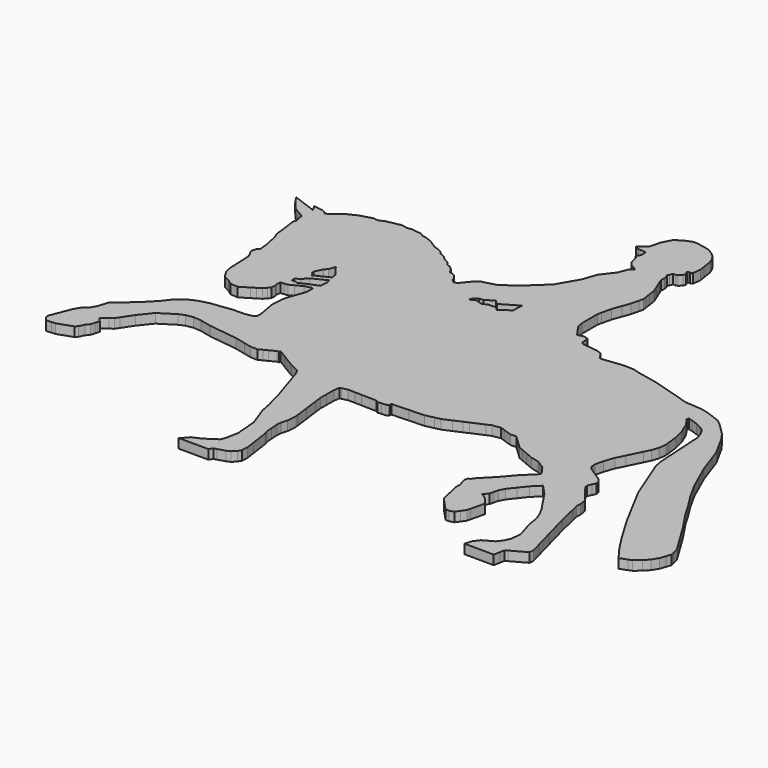
from build123d import *

# Parameters (mm, degrees)
F1_DEPTH = 6.35
F2_SCALE = 0.85


# Not quite as in the source:
# - ends of sketch curves that miss each other by under 0.0002 mm in the source are joined


with BuildPart() as f1:
    # F0 (on Top) → F1 (new body)
    with BuildSketch(Plane.XY):
        Polygon((-13.5594852, 161.1981282), (-15.3749502, 153.9993872), (-17.5161448, 152.6285238), (-20.7511396, 149.630257), (-18.0455062, 148.39569), (-12.6456948, 147.858353), (-12.6219966, 147.147788), (-12.5753876, 145.7501784), (-12.5165612, 143.986504), (-13.7517632, 142.1640286), (-14.1046708, 140.9294616), (-12.911709, 140.0959606), (-12.697206, 139.238355), (-12.2184922, 137.3244142), (-11.4538506, 134.2673718), (-9.3327474, 131.4925488), (-6.5719198, 130.034538), (-4.747133, 129.070862), (-5.6896508, 128.3296646), (-7.3535286, 127.0211836), (-8.5178646, 124.0731326), (-10.0039678, 120.3103004), (-12.3753626, 117.2887926), (-14.3408654, 114.7844288), (-16.4336984, 112.1178606), (-18.105247, 107.3182004), (-19.8354696, 102.3500366), (-23.1120442, 96.7057756), (-27.8045418, 88.6224542), (-31.3029346, 85.3369896), (-40.0668744, 77.1065006), (-50.4377452, 69.6153294), (-54.205886, 68.6302666), (-59.3993478, 67.2725604), (-62.914403, 64.9672056), (-65.692909, 61.5112308), (-68.3397414, 58.2190352), (-70.5160134, 57.337198), (-72.8844364, 59.4073234), (-73.4137978, 61.2885744), (-75.1195348, 63.6401318), (-77.8251682, 65.0510764), (-79.5897316, 65.4038316), (-81.0095662, 68.1746414), (-83.2446646, 70.173469), (-85.5973904, 71.1141072), (-87.1855, 73.1717358), (-90.617294, 74.9848132), (-91.067509, 75.4057166), (-92.902786, 77.1215374), (-96.8436214, 79.0027884), (-97.667064, 80.2373808), (-101.2549918, 82.1186318), (-103.7253704, 82.8240914), (-109.976412, 86.8835956), (-114.0937012, 88.3533158), (-116.6228808, 88.7648466), (-118.9168056, 90.2933678), (-126.0926358, 91.175205), (-128.5630144, 90.7048986), (-132.8142886, 91.5578306), (-136.8693732, 90.7192496), (-139.5204474, 90.171016), (-142.9319214, 89.4655564), (-146.033617, 87.949405), (-147.2354434, 88.046814), (-149.7287074, 88.2489472), (-153.4701782, 87.1649768), (-157.528641, 85.9892108), (-164.1585236, 82.827876), (-166.1786618, 81.272888), (-171.2958728, 77.3340084), (-173.1780636, 76.3345946), (-174.4132402, 77.7455392), (-176.8247924, 78.6861774), (-182.8242724, 79.6855912), (-180.4715212, 75.629135), (-196.5877704, 81.5668422), (-192.9998426, 76.3345946), (-188.2943656, 70.9259948), (-180.8160976, 66.625216), (-180.52161, 63.493523), (-179.698142, 61.6710476), (-180.3883108, 58.723657), (-179.9922486, 55.6745394), (-178.6976106, 45.707681), (-178.5211314, 43.0033684), (-176.7565934, 38.1826516), (-174.9891598, 29.5782492), (-174.3421456, 23.4641644), (-175.8714288, 21.759291), (-176.8125242, 18.7022486), (-173.9942164, 13.167614), (-173.8757254, 10.4908858), (-173.572043, 3.6312094), (-173.2779364, -3.0119828), (-172.4848468, -7.733919), (-170.7487568, -10.5370122), (-169.2194736, -13.0061462), (-165.3238502, -14.8990304), (-161.9123762, -17.485741), (-156.7532552, -17.8927506), (-150.9220502, -14.3583914), (-148.0312508, -12.6062486), (-145.3319928, -10.9701838), (-143.6198804, -8.9613232), (-142.267051, -7.374001), (-141.9729444, -4.5521118), (-142.5023312, -2.7296618), (-142.1407114, 0.0580898), (-139.7966724, 0.3273806), (-137.3711756, 0.606044), (-134.2089264, 2.2674326), (-129.6211022, 4.677791), (-125.033278, 5.7947814), (-124.20981, 5.4420516), (-124.5156006, 0.0899668), (-126.978664, -6.9225922), (-128.9196812, -12.4487686), (-129.8023058, -21.8769184), (-127.5066538, -35.0687894), (-127.6831076, -37.6555254), (-129.3300182, -39.007669), (-134.682484, -39.8895062), (-142.5683712, -40.0267678), (-148.3478364, -40.7748232), (-156.5235884, -41.833038), (-162.2289618, -43.3027582), (-166.6403322, -45.0664326), (-170.22826, -47.2416378), (-174.2867228, -50.710211), (-178.2987036, -55.8449226), (-184.8863714, -62.723268), (-193.3650692, -70.3360544), (-198.4905098, -74.3402374), (-199.3057228, -76.9204456), (-200.7173532, -81.3884326), (-203.0789944, -85.5258894), (-206.431642, -88.4065542), (-208.798033, -92.3547302), (-211.19592, -98.4595186), (-214.3132874, -106.3960788), (-214.19566, -108.2185288), (-211.7847682, -111.206915), (-208.3726592, -110.9816424), (-205.5935944, -110.7981528), (-195.653279, -107.2707786), (-194.2326316, -105.7961054), (-192.585721, -102.3275322), (-190.6311402, -99.917504), (-189.8298972, -97.3421726), (-189.3507008, -95.801942), (-188.9049054, -94.369001), (-189.7036084, -93.4503592), (-191.4109202, -91.4866852), (-187.4030796, -88.4413776), (-185.1084436, -86.69782), (-183.3985664, -84.1324962), (-178.5717028, -76.8906514), (-171.9197984, -68.5932842), (-161.61512, -62.0641126), (-158.0271922, -60.4768158), (-153.2629142, -59.6537542), (-147.7927956, -60.065285), (-140.1283456, -61.8401354), (-120.6822326, -64.2982966), (-113.6962166, -65.9645874), (-108.5202046, -67.1991544), (-103.819579, -67.2790628), (-101.1929904, -65.9473916), (-98.4452946, -64.5543286), (-94.3868318, -62.4967), (-93.0928288, -62.4379244), (-92.7708584, -61.3130092), (-86.8513122, -64.9144244), (-78.7343866, -69.8527178), (-72.2020146, -73.1011238), (-70.6466202, -75.7986546), (-67.0811206, -86.8151426), (-62.3731036, -101.3617734), (-59.1379818, -113.8447812), (-57.9923148, -120.0834022), (-54.3089592, -130.1536386), (-52.9630132, -133.8334382), (-52.5443958, -138.8544594), (-51.7358122, -148.5531446), (-52.5432782, -152.6360168), (-53.5432, -157.6918868), (-54.6103302, -160.1483462), (-57.2334136, -161.8852236), (-59.601481, -163.4532418), (-62.5777768, -165.4240024), (-65.4833336, -166.6866618), (-68.188967, -167.8624278), (-70.0711578, -169.8024798), (-70.8357994, -171.2134244), (-72.1886288, -171.918884), (-72.8356176, -172.7419456), (-52.5753838, -172.7960222), (-51.0100834, -170.5091332), (-49.0462824, -169.9153574), (-44.1587636, -168.43756), (-41.5707576, -167.2617686), (-39.2153648, -164.8360432), (-37.9213618, -162.660838), (-37.6275346, -158.512129), (-38.5710176, -151.8843292), (-40.2222716, -140.2848858), (-41.1129734, -137.546715), (-41.3986472, -133.4065404), (-41.7515548, -128.2918694), (-41.5762948, -125.0391962), (-40.2822918, -120.923939), (-39.8046194, -114.6921252), (-40.0651218, -112.6588552), (-41.2047436, -103.764334), (-42.3415968, -94.8914536), (-42.9747934, -89.9495534), (-42.9297846, -84.9560658), (-42.8709582, -78.4304502), (-42.2566338, -74.5899702), (-41.1064202, -74.3152184), (-37.3378984, -73.4149916), (-32.6724518, -73.5141786), (-28.145486, -73.6104192), (-17.7279554, -73.8318818), (-17.4853346, -74.0242614), (-16.45666, -74.8400332), (-13.720953, -74.6121698), (-10.8976922, -74.3769912), (-9.368409, -73.495154), (-9.0692986, -71.9237068), (2.2961092, -71.495539), (12.4181616, -71.1142088), (18.1943756, -69.8443866), (22.0813122, -68.9899052), (27.76601, -66.4898848), (32.939482, -64.2146798), (36.3673136, -62.7071898), (44.6301114, -59.0733642), (47.571025, -57.7799962), (53.1573486, -56.9123068), (55.8745644, -57.8450202), (61.6975906, -59.8438478), (65.569719, -59.6190578), (66.2569414, -60.2732856), (68.4092358, -62.322202), (74.9568986, -68.5553874), (77.6381734, -69.674486), (81.88833, -71.4483966), (87.2407958, -73.6823774), (92.647262, -74.9761264), (95.4165478, -76.6806442), (98.2669612, -78.4350984), (99.777804, -80.516603), (101.9541014, -83.5148444), (102.6673334, -85.4077032), (101.7776476, -86.2779326), (94.2413152, -93.6494952), (86.9478322, -102.1151374), (78.9430222, -110.3117428), (76.8255512, -113.133632), (75.9811282, -113.0547396), (75.649201, -114.1330458), (75.1786406, -115.661567), (77.1196578, -122.2459582), (76.6021328, -123.4571572), (78.8841958, -134.062597), (79.9635942, -139.078843), (80.8085506, -139.9872486), (81.2150776, -140.4243318), (83.2315328, -142.5922218), (86.1869752, -145.7696348), (88.5441968, -148.3038944), (91.0734018, -148.36267), (93.9496216, -147.4582268), (95.8965062, -144.7177446), (97.9189812, -141.8708364), (98.4967042, -139.4701046), (100.7802658, -129.9807662), (99.6133898, -128.5154148), (97.3194904, -125.63475), (93.6708058, -123.0925656), (92.7147752, -122.6612736), (93.3767246, -121.9167742), (95.3337438, -119.715661), (95.9059042, -117.3900116), (96.7881732, -113.8038618), (98.6735898, -110.2226396), (102.493572, -105.3969952), (106.7284886, -100.047171), (111.9280718, -94.9476638), (114.0244608, -97.1812636), (118.142512, -101.568885), (123.7943168, -110.0118958), (128.3279374, -116.7845264), (130.798316, -121.4288656), (132.7393332, -126.6023122), (133.9188584, -134.093458), (137.4859074, -145.926429), (137.0386134, -149.6946206), (136.6268794, -153.1631938), (134.803515, -157.0432724), (132.278501, -160.282636), (128.804035, -162.27552), (125.0928918, -164.404167), (124.039757, -165.8616698), (122.3109822, -168.2542482), (121.451751, -171.152693), (120.9811906, -172.7400152), (140.876909, -172.893482), (141.647291, -168.6630358), (142.2295606, -165.4655822), (143.8823894, -164.547804), (153.9403322, -158.9628266), (154.2497296, -155.9990022), (152.3248414, -148.8355672), (148.6990422, -135.3422236), (144.2629576, -118.8333666), (141.4003014, -106.378502), (140.4003796, -102.0280916), (140.5951468, -99.0048312), (140.1629404, -96.4833986), (139.7758698, -94.2253132), (136.338564, -89.83726), (130.3979104, -82.253455), (130.0159706, -80.260952), (131.2779188, -77.5280898), (132.3366416, -75.235308), (132.0425604, -72.9425262), (129.9662374, -70.5225666), (125.6313464, -67.710304), (120.1579512, -64.1594094), (118.3345868, -61.749051), (118.0993066, -58.574432), (119.3933096, -52.9894546), (121.7419968, -46.347126), (124.580523, -40.5940514), (129.105533, -31.4229242), (131.2229786, -27.1313148), (132.7522618, -22.6045268), (133.3612522, -17.6188624), (133.0468256, -14.9502114), (132.2212748, -7.9437738), (130.5054794, -0.8137906), (128.9862546, 2.8734258), (127.4524756, 6.5959736), (125.0454192, 10.104501), (123.6337888, 12.1621296), (124.0930716, 13.4510018), (126.6923298, 12.632436), (130.9860728, 11.2802924), (135.5739224, 8.9875106), (137.8166916, 7.0895972), (140.110591, 3.2683196), (141.3658844, -0.9285478), (141.5890488, -4.75742), (142.0390098, -12.4779532), (142.9332168, -27.821001), (143.2861498, -33.8762848), (144.3800516, -39.845361), (148.819743, -51.0711958), (156.1292026, -69.5532772), (164.4222518, -85.1556336), (171.3700916, -98.2271086), (181.7329106, -115.592987), (187.9088444, -125.2344206), (194.9733464, -134.810119), (199.848978, -132.9358022), (202.1429028, -132.053965), (206.3217616, -128.573784), (209.439129, -125.2815884), (211.967191, -121.1609972), (213.2169472, -117.4032704), (214.3132874, -114.1068076), (213.7388664, -111.5767898), (212.8828102, -107.806236), (208.6443884, -100.8661178), (199.5825066, -86.027895), (197.2842384, -82.5810134), (191.0201666, -73.1863408), (187.0080842, -66.2111452), (180.745638, -56.319039), (174.3556838, -44.7984626), (170.5052216, -36.1900724), (166.169975, -26.497915), (162.0055942, -14.6172428), (159.5699374, -7.6684886), (158.4496196, -5.6369458), (156.0258754, -1.2418568), (154.554555, 1.4261846), (151.9164602, 6.2099444), (148.5511888, 10.7893866), (143.8720516, 15.3919428), (140.1312158, 19.0715646), (137.1780848, 21.2618066), (131.8384968, 23.2406698), (127.4190238, 24.878538), (122.4318608, 25.9900928), (116.823109, 26.4206482), (111.2171766, 26.8510004), (105.2568888, 28.6497522), (94.0084226, 32.0444368), (84.3141062, 34.970085), (78.2545298, 36.2179362), (70.9920856, 37.7135136), (66.2295602, 39.1155682), (63.1462796, 39.202487), (58.917459, 39.3216892), (54.8880538, 38.8593076), (50.1211088, 38.3122678), (44.488862, 37.665914), (42.5732448, 40.198294), (40.6840182, 42.6957998), (37.0634768, 43.825033), (31.9443862, 44.4329312), (26.9290546, 45.0285358), (25.6531872, 46.3983324), (25.2889512, 49.7535708), (25.1190506, 51.3188458), (23.7495842, 51.6892286), (21.7927174, 52.2184884), (19.8763636, 51.639597), (18.151602, 51.1185922), (14.9603206, 55.6102012), (12.5271276, 59.0348324), (11.6393468, 63.5017272), (11.6393468, 66.8265618), (11.6393468, 68.1121574), (11.6393468, 76.693395), (12.231751, 79.2636464), (13.7633202, 85.9085404), (15.940151, 91.8542994), (17.8449732, 97.0570576), (19.124041, 102.2202934), (19.8395082, 105.108502), (19.4781932, 107.6610496), (18.926302, 111.559848), (18.2781702, 116.1385282), (16.6403274, 120.1439812), (14.4763236, 125.436249), (13.451713, 127.9420606), (13.6913874, 130.6541456), (13.2335778, 133.0074302), (12.4737622, 134.1599298), (13.1893818, 135.7156798), (14.0614146, 137.611358), (16.0452562, 137.611358), (17.0764962, 138.0032292), (18.8621924, 139.8475232), (19.6955156, 141.6323558), (18.4455308, 143.5361366), (18.4455308, 144.3095666), (20.2312016, 144.3095666), (21.6597738, 145.0234844), (22.3461834, 150.2638092), (21.7788236, 153.9475204), (20.8241392, 160.145857), (19.4551046, 163.7749582), (17.6694084, 166.3926822), (14.6337274, 169.069893), (10.4927908, 171.2421264), (6.633718, 171.9813426), (1.8718784, 172.8934566), (-0.3786378, 172.8934566), (-3.0685486, 171.8623436), (-6.073267, 170.7105552), (-8.4256372, 168.9471602), (-10.3303578, 167.5193246), (-11.7440456, 164.9462284), align=None)
        Polygon((-138.7489986, 5.6613552), (-139.179808, 8.173212), (-135.9486994, 10.0391468), (-133.0047886, 13.4121906), (-123.5268802, 18.148808), (-122.8088476, 15.924022), (-123.024265, 10.3979726), (-131.9995582, 6.737858), (-134.5126342, 5.230749), (-136.2358972, 5.876671), align=None, mode=Mode.SUBTRACT)
        Polygon((-124.3166932, 21.6653872), (-134.2972422, 16.7852344), (-134.58444, 18.5076338), (-135.733282, 18.7229242), (-136.1640914, 20.8041748), (-133.5792096, 26.0431534), (-131.7123604, 27.9808686), (-130.2762952, 32.2868798), (-126.6143772, 27.406727), (-124.7877616, 24.9724418), align=None, mode=Mode.SUBTRACT)
        Polygon((-37.1232684, 52.489608), (-25.48128, 59.343798), (-25.9597398, 52.064539), (-32.9105461572, 46.9561600662), (-35.103181, 49.0890814), (-40.6317958, 48.929671), (-43.5555644, 47.3356686), (-49.031017, 49.0890814), (-51.1042412, 47.4419422), (-52.592732, 47.6013272), (-48.4462582, 51.3738114), (-45.6819762, 51.5331964), (-40.1001992, 55.0399966), align=None, mode=Mode.SUBTRACT)
    extrude(amount=F1_DEPTH)


with BuildPart() as f1_1:
    # F2: moved
    add(f1.part.scale(F2_SCALE).moved(Location((-0.46028229, 25.77935154, 0.9525))))


solid = f1_1.part
